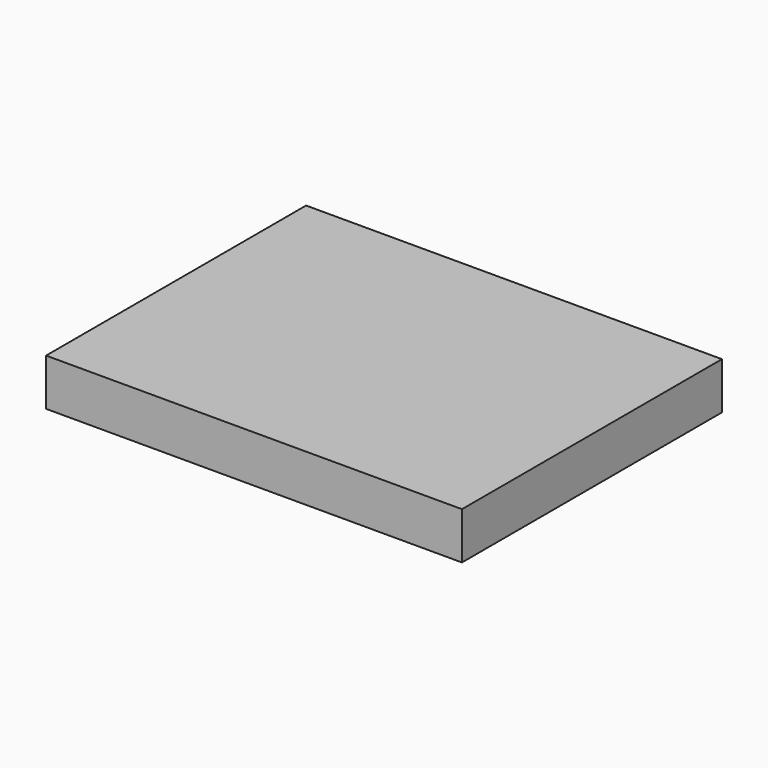
from build123d import *

# Parameters (mm, degrees)
F0_W     = 112.5728
F0_H     = 87.9652537405
F1_DEPTH = 12.7


# Not quite as in the source:
# - the program builds the solid bodies; features that only make, move or delete a surface that nothing else refers to are left out


with BuildPart() as f1:
    # F0 (on Top) → F1 (new body)
    with BuildSketch(Plane.XY):
        with Locations((0.3974718951, 8.2319211215)):
            Rectangle(F0_W, F0_H)
    extrude(amount=-F1_DEPTH)


solid = f1.part
